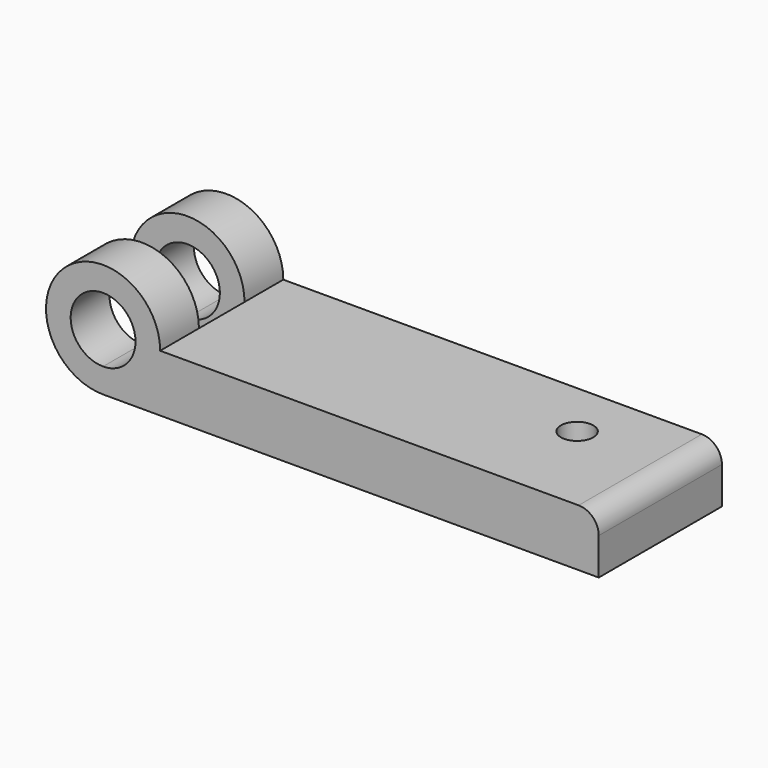
from build123d import *

# Parameters (mm, degrees)
F1_DEPTH = 30.1625
F2_DEPTH = 30.1625
F3_W     = 44.704
F3_H     = 22.3266
F4_DEPTH = 30.1625
F5_R     = 6.35
F6_DEPTH = 22.352


with BuildPart() as f1:
    # F0 (on Front) → F1 (new body, symmetric)
    with BuildSketch(Plane.XZ):
        with BuildLine():
            ThreePointArc((22.352, 0), (15.805251, -15.805251), (0, -22.352))
            Line((0, -22.352), (194.2084, -22.352))
            Line((194.2084, -22.352), (194.2084, -7.874))
            ThreePointArc((194.2084, -7.874), (191.902159, -2.306241), (186.3344, 0))
            Line((186.3344, 0), (22.352, 0))
        make_face()
    extrude(amount=F1_DEPTH, both=True)

    # F0 (on Front) → F2 (join, symmetric)
    with BuildSketch(Plane.XZ):
        with BuildLine():
            ThreePointArc((22.352, 0), (-15.805251, 15.805251), (0, -22.352))
            ThreePointArc((0, -22.352), (15.805251, -15.805251), (22.352, 0))
        make_face()
        with BuildLine():
            ThreePointArc((0, -12.7), (-8.980256, 8.980256), (12.7, 0))
            ThreePointArc((12.7, 0), (8.980256, -8.980256), (0, -12.7))
        make_face(mode=Mode.SUBTRACT)
    extrude(amount=F2_DEPTH, both=True)

    # F3 (on Top) → F4 (cut, symmetric)
    with BuildSketch(Plane.XY):
        Rectangle(F3_W, F3_H)
    extrude(amount=F4_DEPTH, both=True, mode=Mode.SUBTRACT)

    # F5 (on face) → F6 (cut)
    with BuildSketch(Plane.XY):
        with Locations((155.3464, 7.8105)):
            Circle(F5_R)
    extrude(amount=-F6_DEPTH, mode=Mode.SUBTRACT)


solid = f1.part
